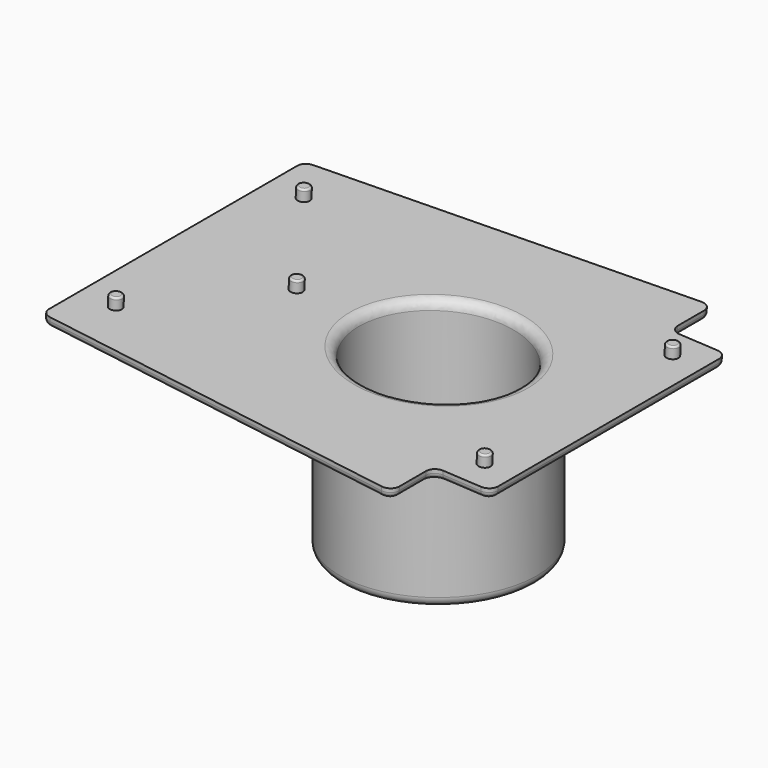
from build123d import *

# Parameters (mm, degrees)
F3_DEPTH  = 2.5
F4_R      = 2.5
F5_R      = 1.5
F6_R      = 26
F6_R_2    = 21
F7_DEPTH  = 50
F9_DEPTH  = 10
F11_DEPTH = 17
F12_R     = 2.49999
F13_R     = 5
F14_R     = 1.625
F15_DEPTH = 3
F16_R     = 0.5


# Not quite as in the source:
# - a fillet or chamfer is up to 0.001 mm smaller than in the source, because OpenCascade refuses the exact size


with BuildPart() as f3:
    # F2 (on line) → F3 (new body)
    with BuildSketch(Plane(origin=(0, 0, 0), x_dir=(0.9987523434, 0, -0.0499375258), z_dir=(-0.0499375258, 0, -0.9987523434))):
        Polygon((100, 53.0810991168), (0, 43.405495584), (0, -43.0531017482), (100, -53.0106203496), (100, -39), (115, -39), (115, 39), (100, 39), align=None)
    extrude(amount=F3_DEPTH)

    # F4
    f4_edges = [f3.edges().sort_by_distance(p)[0] for p in [
        (-0.062422, -43.405496, -1.24844),
        (-0.062422, 43.053102, -1.24844),
        (114.794098, 39, -6.991256),
        (99.812812, 53.01062, -6.242193),
        (99.812812, 39, -6.242193),
        (114.794098, -39, -6.991256),
        (99.812812, -53.081099, -6.242193),
        (99.812812, -39, -6.242193),
    ]]
    fillet(f4_edges, radius=F4_R)

    # F5
    f5_edges = [f3.edges().sort_by_distance(p)[0] for p in [
        (114.731676, 0, -8.239696),
        (-0.124844, -0.173017, -2.496881),
        (99.750391, -45.913767, -7.490633),
        (99.750391, 45.874659, -7.490633),
        (49.565369, 48.007195, -4.981387),
        (49.572308, -48.220002, -4.981734),
        (107.241033, -39, -7.865165),
        (107.241033, 39, -7.865165),
    ]]
    fillet(f5_edges, radius=F5_R)


with BuildPart() as f7:
    # F6 (on Top) → F7 (new body)
    with BuildSketch(Plane.XY):
        with Locations((69.91, 0)):
            Circle(F6_R)
        with Locations((69.91, 0)):
            Circle(F6_R_2, mode=Mode.SUBTRACT)
    extrude(amount=-F7_DEPTH)


with BuildPart() as f3_1:
    add(f3.part)

    # F8: union F7
    add(f7.part)

    # F6 (on Top) → F9 (cut)
    with BuildSketch(Plane.XY):
        with Locations((69.91, 0)):
            Circle(F6_R_2)
    extrude(amount=-F9_DEPTH, mode=Mode.SUBTRACT)

    # F10 (on face) → F11 (cut)
    with BuildSketch(Plane(origin=(0, 0, 0), x_dir=(0.9987523434, 0, -0.0499375258), z_dir=(0.0499375258, 0, 0.9987523434))):
        with BuildLine():
            add(Edge.make_bspline(
                [(43.4973326317, 0), (43.4973326317, -45.1440074052), (83.2473326317, -22.5720037026), (122.9973326317, 0), (83.2473326317, 22.5720037026), (43.4973326317, 45.1440074052), (43.4973326317, 0)],
                knots=[0, 0, 0, 2.0943951024, 2.0943951024, 4.1887902048, 4.1887902048, 6.2831853072, 6.2831853072, 6.2831853072], degree=2, weights=[1, 0.5, 1, 0.5, 1, 0.5, 1]))
        make_face()
    extrude(amount=F11_DEPTH, mode=Mode.SUBTRACT)

    # F12 (radius 2.5 in the source; OpenCascade refuses exactly that, so slightly less here)
    f12_edges = [f3_1.edges().sort_by_distance(p)[0] for p in [
        (43.91, 0, -50),
        (48.91, 0, -50),
        (48.91, 0, -2.445496),
    ]]
    fillet(f12_edges, radius=F12_R)

    # F13
    f13_edges = [f3_1.edges().sort_by_distance(p)[0] for p in [
        (43.91, 0, -4.698619),
    ]]
    fillet(f13_edges, radius=F13_R)

    # F14 (on face) → F15 (join)
    with BuildSketch(Plane(origin=(0, 0, 0), x_dir=(0.9987523434, 0, -0.0499375258), z_dir=(0.0499375258, 0, 0.9987523434))):
        with Locations((107, 31)):
            Circle(F14_R)
        with Locations((107, -31)):
            Circle(F14_R)
        with Locations((9.5225282311, 31)):
            Circle(F14_R)
        with Locations((9.5225282311, -31)):
            Circle(F14_R)
        with Locations((32.4829758469, 0)):
            Circle(F14_R)
    extrude(amount=F15_DEPTH)

    # F16
    f16_edges = [f3_1.edges().sort_by_distance(p)[0] for p in [
        (105.393341, 31, -2.26591),
        (105.393341, -31, -2.26591),
        (30.969288, 0, 1.455286),
        (8.037487, 31, 2.601874),
        (8.037487, -31, 2.601874),
    ]]
    fillet(f16_edges, radius=F16_R)


solid = f3_1.part
